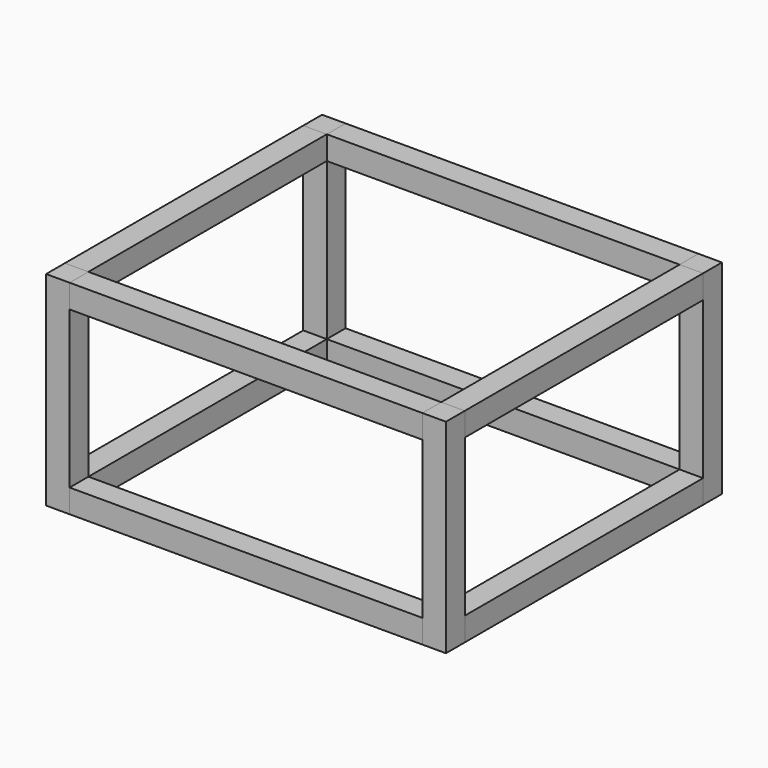
from build123d import *

# Parameters (mm, degrees)
F0_W     = 571.5
F0_H     = 38.1
F1_DEPTH = 38.1
F0_W_2   = 38.1
F0_H_2   = 482.6
F3_W     = 38.1
F3_H     = 38.1
F4_DEPTH = 165.1


# Not quite as in the source:
# - a pattern or mirror of a feature is missing from the dataset's text; its kind, count and spacing are read off the source's solid


with BuildPart() as f1:
    # F0 (on Top) → F1 (new body)
    with BuildSketch(Plane.XY):
        with Locations((0, 260.35)):
            Rectangle(F0_W, F0_H)
    extrude(amount=F1_DEPTH)


with BuildPart() as f1b:
    # F0 (on Top) → F1, piece 2 (new body)
    with BuildSketch(Plane.XY):
        with Locations((-304.8, 0)):
            Rectangle(F0_W_2, F0_H_2)
    extrude(amount=F1_DEPTH)


with BuildPart() as f1c:
    # F0 (on Top) → F1, piece 3 (new body)
    with BuildSketch(Plane.XY):
        with Locations((304.8, 0)):
            Rectangle(F0_W_2, F0_H_2)
    extrude(amount=F1_DEPTH)


with BuildPart() as f1d:
    # F0 (on Top) → F1, piece 4 (new body)
    with BuildSketch(Plane.XY):
        with Locations((0, -260.35)):
            Rectangle(F0_W, F0_H)
    extrude(amount=F1_DEPTH)


with BuildPart() as f1_copies_1:
    # F1_copies: instance of F1
    add(f1.part.mirror(Plane.XY.offset(165.1)))


with BuildPart() as f1_2_copies_1:
    # F1_2_copies: instance of F1b
    add(f1b.part.mirror(Plane.XY.offset(165.1)))


with BuildPart() as f1_3_copies_1:
    # F1_3_copies: instance of F1c
    add(f1c.part.mirror(Plane.XY.offset(165.1)))


with BuildPart() as f1_4_copies_1:
    # F1_4_copies: instance of F1d
    add(f1d.part.mirror(Plane.XY.offset(165.1)))


with BuildPart() as f4:
    # F3 (on offset) → F4 (new body, symmetric)
    with BuildSketch(Plane.XY.offset(165.1)):
        with Locations((-304.8, -260.35)):
            Rectangle(F3_W, F3_H)
    extrude(amount=F4_DEPTH, both=True)


with BuildPart() as f4b:
    # F3 (on offset) → F4, piece 2 (new body, symmetric)
    with BuildSketch(Plane.XY.offset(165.1)):
        with Locations((304.8, -260.35)):
            Rectangle(F3_W, F3_H)
    extrude(amount=F4_DEPTH, both=True)


with BuildPart() as f4c:
    # F3 (on offset) → F4, piece 3 (new body, symmetric)
    with BuildSketch(Plane.XY.offset(165.1)):
        with Locations((304.8, 260.35)):
            Rectangle(F3_W, F3_H)
    extrude(amount=F4_DEPTH, both=True)


with BuildPart() as f4d:
    # F3 (on offset) → F4, piece 4 (new body, symmetric)
    with BuildSketch(Plane.XY.offset(165.1)):
        with Locations((-304.8, 260.35)):
            Rectangle(F3_W, F3_H)
    extrude(amount=F4_DEPTH, both=True)


solid = Compound([f1.part, f1b.part, f1c.part, f1d.part, f1_copies_1.part, f1_2_copies_1.part, f1_3_copies_1.part, f1_4_copies_1.part, f4.part, f4b.part, f4c.part, f4d.part])
